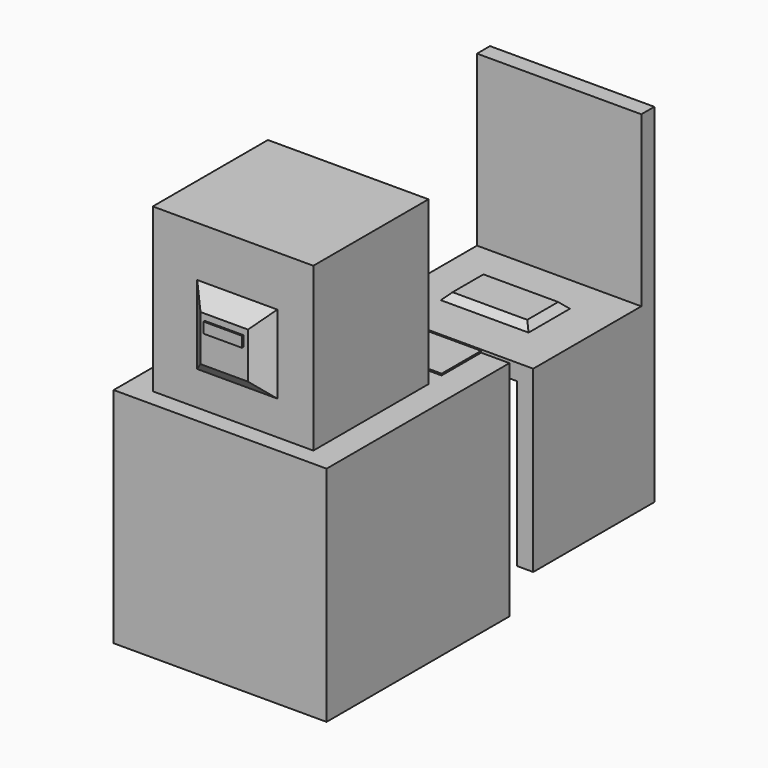
from build123d import *

# Parameters (mm, degrees)
F0_W          = 25.6471270695
F0_H          = 28.9241932333
F1_DEPTH      = 23.622
F2_T          = -2.54
F3_DEPTH      = 25.4
F4_T          = 2.54
F4_T3_DEPTH   = 30.7271270695
F5_W          = 33.229653025
F5_H          = 35.672545433
F6_DEPTH      = 25.4
F7_DEPTH      = 9.398
F8_T          = -2.54
F9_W          = 25.0606182963
F9_H          = 22.4626017734
F10_DEPTH     = 25.4
F11_W         = 17.3738580197
F11_H         = 16.2390768528
F12_DEPTH     = 0.254
F13_W         = 20.8540516905
F13_H         = 7.7100452036
F14_DEPTH     = 0.254
F15_W         = 17.5806907937
F15_H         = 17.3154473305
F16_DEPTH     = 2.54
F17_T4_DEPTH  = 43.7089899514
F17_T9_DEPTH  = 30.3795969093
F17_T14_DEPTH = 43.7089899514
F17_T19_DEPTH = 30.3795969093
F18_W         = 6.000591442
F18_H         = 1.6524102539
F19_DEPTH     = 0.254
F20_W         = 2.1683480591
F20_H         = 3.2685222104
F21_DEPTH     = 0.762
F22_W         = 21.8256991357
F22_H         = 16.1863591056
F23_DEPTH     = 1.016
F24_W         = 11.2391430885
F24_H         = 19.774777656
F25_DEPTH     = 8.382
F26_W         = 2.0196139812
F26_H         = 1.8313727342
F27_DEPTH     = 0.508
F28_W         = 4.9204975367
F28_H         = 1.1510411277
F29_DEPTH     = 0.508
F30_W         = 4.5765712857
F30_H         = 0.9553717311
F31_DEPTH     = 0.508
F32_W         = 6.3235126436
F32_H         = 2.8299971759
F33_DEPTH     = 2.6162
F34_W         = 0.9528808296
F34_H         = 0.6592851132
F35_DEPTH     = 0.2032
F36_T4_DEPTH  = 47.9539982934
F36_T9_DEPTH  = 29.2505086845
F36_T14_DEPTH = 47.9539982934
F36_T19_DEPTH = 29.2505086845
F37_W         = 0.83655864
F37_H         = 0.8337534964
F38_DEPTH     = 0.508
F37_W_2       = 0.7356256247
F37_H_2       = 0.5238540471
F37_W_3       = 1.1432357132
F37_H_3       = 0.6819479167
F37_W_4       = 0.7289908826
F37_H_4       = 0.5421712995
F37_W_5       = 1.2829229236
F37_H_5       = 0.4794821143
F37_W_6       = 0.6956644356
F37_H_6       = 0.5608797073
F37_W_7       = 1.0760016739
F37_H_7       = 0.4885531962
F37_W_8       = 0.6218552589
F37_H_8       = 0.4100985825
F37_W_9       = 0.7822141051
F37_H_9       = 0.4685148597
F37_W_10      = 1.0629147291
F37_H_10      = 0.598076731
F37_W_11      = 1.1558197439
F37_H_11      = 0.371992588
F37_W_12      = 0.8621029556
F37_H_12      = 0.3762468696
F37_W_13      = 0.7478930056
F37_H_13      = 0.5268156528
F37_W_14      = 1.0761059821
F37_H_14      = 0.5310699344


# Not quite as in the source:
# - a fillet or chamfer that OpenCascade refuses, or shapes differently, is made with other operations: its cross-section is extruded or revolved along the edge and cut away or added
# - a shell that OpenCascade refuses in one call is made with other operations: the cavity is built on its own and cut out


with BuildPart() as f1:
    # F0 (on Front) → F1 (new body)
    with BuildSketch(Plane.XZ):
        with Locations((-20.8924110048, 14.4620966166)):
            Rectangle(F0_W, F0_H)
    extrude(amount=-F1_DEPTH)

    # F2
    f2_openings = [f1.faces().sort_by_distance(p)[0] for p in [
        (-33.715975, 11.811, 14.462097),
        (-20.892411, 11.811, 28.924193),
        (-20.892411, 0, 14.462097),
        (-8.068847, 11.811, 14.462097),
    ]]
    offset(amount=F2_T, openings=f2_openings)

    # F3 (add): a face of the model
    f3_faces = [f1.faces().sort_by_distance(p)[0] for p in [
        (-20.8924110048, 11.811, 0),
    ]]
    extrude(f3_faces, amount=F3_DEPTH)

    # F4: shell of thickness 2.54, made by hand


with BuildPart() as f4_core1:
    # F4_t2: copy of F1
    add(f1.part)

    # the walls: a layer under each face that stays
    f4_faces = [f4_core1.faces().sort_by_distance(p)[0] for p in [
        (-8.06884747, 11.811, 1.7620966166),
        (-20.8924110048, 10.541, 2.54),
        (-20.8924110048, 21.082, 15.7320966166),
        (-33.7159745395, 11.811, 1.7620966166),
        (-20.8924110048, 22.352, 28.9241932333),
    ]]
    thicken(f4_faces, amount=-F4_T, mode=Mode.SUBTRACT)

    # F4_s4 → F4_t3 (cut)
    with BuildSketch(Plane.YZ.offset(-36.2559745395)):
        Polygon((21.0566, 2.5654), (21.082, 0), (23.622, 0), (23.622, 2.54), align=None)
    extrude(amount=F4_T3_DEPTH, mode=Mode.SUBTRACT)


with BuildPart() as f1_1:
    add(f1.part)

    # what is left inside the walls is the cavity
    f4_cavity = [f4_core1.part.solids().sort_by_distance(p)[0] for p in [
        (-31.150575, 15.748, -12.7),
    ]]
    add(f4_cavity, mode=Mode.SUBTRACT)

    # F22 (on face) → F23 (join)
    with BuildSketch(Plane.XY.offset(2.54)):
        with Locations((-21.3105017319, 11.1090062419)):
            Rectangle(F22_W, F22_H)
    extrude(amount=F23_DEPTH)

    # F36: chamfer of 5.08 on 4 edges, made by hand


with BuildPart() as f6:
    # F5 (on Top) → F6 (new body)
    with BuildSketch(Plane.XY):
        with Locations((-19.6373554645, -28.7940166891)):
            Rectangle(F5_W, F5_H)
    extrude(amount=-F6_DEPTH)

    # F7 (add): a face of the model
    f7_faces = [f6.faces().sort_by_distance(p)[0] for p in [
        (-19.6373554645, -28.7940166891, 0),
    ]]
    extrude(f7_faces, amount=F7_DEPTH)

    # F8
    f8_openings = [f6.faces().sort_by_distance(p)[0] for p in [
        (-19.637355, -28.794017, -25.4),
        (-19.637355, -10.957744, -8.001),
    ]]
    offset(amount=F8_T, openings=f8_openings)

    # F9 (on face) → F10 (join)
    with BuildSketch(Plane.XY.offset(9.398)):
        with Locations((-19.7930010036, -32.6825478114)):
            Rectangle(F9_W, F9_H)
    extrude(amount=F10_DEPTH)

    # F11 (on face) → F12 (join)
    with BuildSketch(Plane(origin=(0, -21.4512469247, 0), x_dir=(-1, 0, 0), z_dir=(0, 1, 0))):
        with Locations((20.0650831684, 20.4758495092)):
            Rectangle(F11_W, F11_H)
    extrude(amount=F12_DEPTH)

    # F13 (on face) → F14 (join)
    with BuildSketch(Plane.XY.offset(9.398)):
        with Locations((-17.8662652615, -14.8127665743)):
            Rectangle(F13_W, F13_H)
    extrude(amount=F14_DEPTH)

    # F15 (on face) → F16 (join)
    with BuildSketch(Plane.XZ.offset(43.9138486981)):
        with Locations((-19.1343412735, 20.8285525441)):
            Rectangle(F15_W, F15_H)
    extrude(amount=F16_DEPTH)

    # F17: chamfer of 5.08 on 4 edges, made by hand


with BuildPart() as f17_tool2:
    # F17_s3 → F17_t4 (new body)
    with BuildSketch(Plane.YZ.offset(2.7201537023)):
        Polygon((-41.3738486981, 29.4862762094), (-46.4538486981, 24.4062762094), (-46.4538486981, 29.4862762094), align=None)
    extrude(amount=-F17_T4_DEPTH)

    split(bisect_by=Plane.XZ.offset(43.9138486981), keep=Keep.TOP)


with BuildPart() as f6_1:
    add(f6.part)

    # F17_t1: cut F17_tool2
    add(f17_tool2.part, mode=Mode.SUBTRACT)


with BuildPart() as f17_tool7:
    # F17_s8 → F17_t9 (new body)
    with BuildSketch(Plane.XY.offset(42.5504257882)):
        Polygon((-27.9246866703, -41.3738486981), (-22.8446866703, -46.4538486981), (-27.9246866703, -46.4538486981), align=None)
    extrude(amount=-F17_T9_DEPTH)

    split(bisect_by=Plane.XZ.offset(43.9138486981), keep=Keep.TOP)


with BuildPart() as f6_2:
    add(f6_1.part)

    # F17_t6: cut F17_tool7
    add(f17_tool7.part, mode=Mode.SUBTRACT)


with BuildPart() as f17_tool12:
    # F17_s13 → F17_t14 (new body)
    with BuildSketch(Plane.YZ.offset(-40.9888362492)):
        Polygon((-41.3738486981, 12.1708288789), (-46.4538486981, 17.2508288789), (-46.4538486981, 12.1708288789), align=None)
    extrude(amount=F17_T14_DEPTH)

    split(bisect_by=Plane.XZ.offset(43.9138486981), keep=Keep.TOP)


with BuildPart() as f6_3:
    add(f6_2.part)

    # F17_t11: cut F17_tool12
    add(f17_tool12.part, mode=Mode.SUBTRACT)


with BuildPart() as f17_tool17:
    # F17_s18 → F17_t19 (new body)
    with BuildSketch(Plane.XY.offset(12.1708288789)):
        Polygon((-10.3439958766, -41.3738486981), (-15.4239958766, -46.4538486981), (-10.3439958766, -46.4538486981), align=None)
    extrude(amount=F17_T19_DEPTH)

    split(bisect_by=Plane.XZ.offset(43.9138486981), keep=Keep.TOP)


with BuildPart() as f6_4:
    add(f6_3.part)

    # F17_t16: cut F17_tool17
    add(f17_tool17.part, mode=Mode.SUBTRACT)

    # F18 (on face) → F19 (join)
    with BuildSketch(Plane.XZ.offset(46.4538486981)):
        with Locations((-19.1577738151, 22.5839214399)):
            Rectangle(F18_W, F18_H)
    extrude(amount=F19_DEPTH)

    # F20 (on face) → F21 (join)
    with BuildSketch(Plane.XY.offset(9.398)):
        with Locations((-30.9085892513, -15.8493197523)):
            Rectangle(F20_W, F20_H)
    extrude(amount=F21_DEPTH)

    # F24 (on face) → F25 (join)
    with BuildSketch(Plane(origin=(-36.252181977, 0, 0), x_dir=(0, -1, 0), z_dir=(-1, 0, 0))):
        with Locations((18.089174293, -15.512611172)):
            Rectangle(F24_W, F24_H)
    extrude(amount=F25_DEPTH)

    # F26 (on face) → F27 (join)
    with BuildSketch(Plane(origin=(0, -12.4696027488, 0), x_dir=(-1, 0, 0), z_dir=(0, 1, 0))):
        with Locations((38.6133119464, -8.2744567189)):
            Rectangle(F26_W, F26_H)
    extrude(amount=F27_DEPTH)

    # F28 (on face) → F29 (join)
    with BuildSketch(Plane(origin=(0, -12.4696027488, 0), x_dir=(-1, 0, 0), z_dir=(0, 1, 0))):
        with Locations((40.4411107302, -13.2004530169)):
            Rectangle(F28_W, F28_H)
    extrude(amount=F29_DEPTH)

    # F30 (on face) → F31 (join)
    with BuildSketch(Plane(origin=(0, -12.4696027488, 0), x_dir=(-1, 0, 0), z_dir=(0, 1, 0))):
        with Locations((40.2691476047, -15.9902970375)):
            Rectangle(F30_W, F30_H)
    extrude(amount=F31_DEPTH)

    # F32 (on face) → F33 (join)
    with BuildSketch(Plane(origin=(-36.252181977, 0, 0), x_dir=(0, -1, 0), z_dir=(-1, 0, 0))):
        with Locations((39.3726844341, -23.985001412)):
            Rectangle(F32_W, F32_H)
    extrude(amount=F33_DEPTH)

    # F34 (on face) → F35 (join)
    with BuildSketch(Plane.XY.offset(-22.5700028241)):
        with Locations((-36.7286223918, -39.0430418774)):
            Rectangle(F34_W, F34_H)
    extrude(amount=F35_DEPTH)


with BuildPart() as f36_tool2:
    # F36_s3 → F36_t4 (new body)
    with BuildSketch(Plane.YZ.offset(2.6664974148)):
        Polygon((19.2021857947, -1.524), (14.1221857947, 3.556), (19.2021857947, 3.556), align=None)
    extrude(amount=-F36_T4_DEPTH)

    split(bisect_by=Plane.XY.offset(2.54), keep=Keep.TOP)


with BuildPart() as f1_2:
    add(f1_1.part)

    # F36_t1: cut F36_tool2
    add(f36_tool2.part, mode=Mode.SUBTRACT)


with BuildPart() as f36_tool7:
    # F36_s8 → F36_t9 (new body)
    with BuildSketch(Plane.XZ.offset(-19.2021857947)):
        Polygon((-32.2233512998, -1.524), (-27.1433512998, 3.556), (-32.2233512998, 3.556), align=None)
    extrude(amount=F36_T9_DEPTH)

    split(bisect_by=Plane.XY.offset(2.54), keep=Keep.TOP)


with BuildPart() as f1_3:
    add(f1_2.part)

    # F36_t6: cut F36_tool7
    add(f36_tool7.part, mode=Mode.SUBTRACT)


with BuildPart() as f36_tool12:
    # F36_s13 → F36_t14 (new body)
    with BuildSketch(Plane.YZ.offset(-45.2875008786)):
        Polygon((3.0158266891, -1.524), (8.0958266891, 3.556), (3.0158266891, 3.556), align=None)
    extrude(amount=F36_T14_DEPTH)

    split(bisect_by=Plane.XY.offset(2.54), keep=Keep.TOP)


with BuildPart() as f1_4:
    add(f1_3.part)

    # F36_t11: cut F36_tool12
    add(f36_tool12.part, mode=Mode.SUBTRACT)


with BuildPart() as f36_tool17:
    # F36_s18 → F36_t19 (new body)
    with BuildSketch(Plane.XZ.offset(10.0483228898)):
        Polygon((-10.3976521641, -1.524), (-15.4776521641, 3.556), (-10.3976521641, 3.556), align=None)
    extrude(amount=-F36_T19_DEPTH)

    split(bisect_by=Plane.XY.offset(2.54), keep=Keep.TOP)


with BuildPart() as f1_5:
    add(f1_4.part)

    # F36_t16: cut F36_tool17
    add(f36_tool17.part, mode=Mode.SUBTRACT)


with BuildPart() as f38:
    # F37 (on Top) → F38 (new body)
    with BuildSketch(Plane.XY):
        Polygon((-47.7759763598, -38.6007763445), (-47.7759763598, -38.0017347634), (-48.7721376121, -38.0017347634), (-48.7721376121, -38.6007763445), (-48.6606992781, -38.6007763445), (-47.8241406381, -38.6007763445), align=None)
        with Locations((-48.2424199581, -39.0176530927)):
            Rectangle(F37_W, F37_H)
    extrude(amount=F38_DEPTH)


with BuildPart() as f38b:
    # F37 (on Top) → F38, piece 2 (new body)
    with BuildSketch(Plane.XY):
        with Locations((-47.1070185304, -37.4404694885)):
            Rectangle(F37_W_2, F37_H_2)
    extrude(amount=F38_DEPTH)


with BuildPart() as f38c:
    # F37 (on Top) → F38, piece 3 (new body)
    with BuildSketch(Plane.XY):
        with Locations((-48.2318531722, -37.4272111803)):
            Rectangle(F37_W_3, F37_H_3)
    extrude(amount=F38_DEPTH)


with BuildPart() as f38d:
    # F37 (on Top) → F38, piece 4 (new body)
    with BuildSketch(Plane.XY):
        with Locations((-47.1084099263, -36.6477929056)):
            Rectangle(F37_W_4, F37_H_4)
    extrude(amount=F38_DEPTH)


with BuildPart() as f38e:
    # F37 (on Top) → F38, piece 5 (new body)
    with BuildSketch(Plane.XY):
        with Locations((-48.2132434845, -36.6469696164)):
            Rectangle(F37_W_5, F37_H_5)
    extrude(amount=F38_DEPTH)


with BuildPart() as f38f:
    # F37 (on Top) → F38, piece 6 (new body)
    with BuildSketch(Plane.XY):
        with Locations((-47.1567194909, -35.9333977103)):
            Rectangle(F37_W_6, F37_H_6)
    extrude(amount=F38_DEPTH)


with BuildPart() as f38g:
    # F37 (on Top) → F38, piece 7 (new body)
    with BuildSketch(Plane.XY):
        with Locations((-48.3284760267, -35.9984207898)):
            Rectangle(F37_W_7, F37_H_7)
    extrude(amount=F38_DEPTH)


with BuildPart() as f38h:
    # F37 (on Top) → F38, piece 8 (new body)
    with BuildSketch(Plane.XY):
        with Locations((-47.1879057586, -39.1126889735)):
            Rectangle(F37_W_8, F37_H_8)
    extrude(amount=F38_DEPTH)


with BuildPart() as f38i:
    # F37 (on Top) → F38, piece 9 (new body)
    with BuildSketch(Plane.XY):
        with Locations((-47.2700297832, -39.9314910173)):
            Rectangle(F37_W_9, F37_H_9)
    extrude(amount=F38_DEPTH)


with BuildPart() as f38j:
    # F37 (on Top) → F38, piece 10 (new body)
    with BuildSketch(Plane.XY):
        with Locations((-48.4051033854, -40.0122273713)):
            Rectangle(F37_W_10, F37_H_10)
    extrude(amount=F38_DEPTH)


with BuildPart() as f38k:
    # F37 (on Top) → F38, piece 11 (new body)
    with BuildSketch(Plane.XY):
        with Locations((-47.4454332143, -40.679089725)):
            Rectangle(F37_W_11, F37_H_11)
    extrude(amount=F38_DEPTH)


with BuildPart() as f38l:
    # F37 (on Top) → F38, piece 12 (new body)
    with BuildSketch(Plane.XY):
        with Locations((-48.5138017684, -40.779016912)):
            Rectangle(F37_W_12, F37_H_12)
    extrude(amount=F38_DEPTH)


with BuildPart() as f38m:
    # F37 (on Top) → F38, piece 13 (new body)
    with BuildSketch(Plane.XY):
        with Locations((-47.1978355199, -41.4876379073)):
            Rectangle(F37_W_13, F37_H_13)
    extrude(amount=F38_DEPTH)


with BuildPart() as f38n:
    # F37 (on Top) → F38, piece 14 (new body)
    with BuildSketch(Plane.XY):
        with Locations((-48.5091153532, -41.5869280696)):
            Rectangle(F37_W_14, F37_H_14)
    extrude(amount=F38_DEPTH)


solid = Compound([f6_4.part, f1_5.part])
